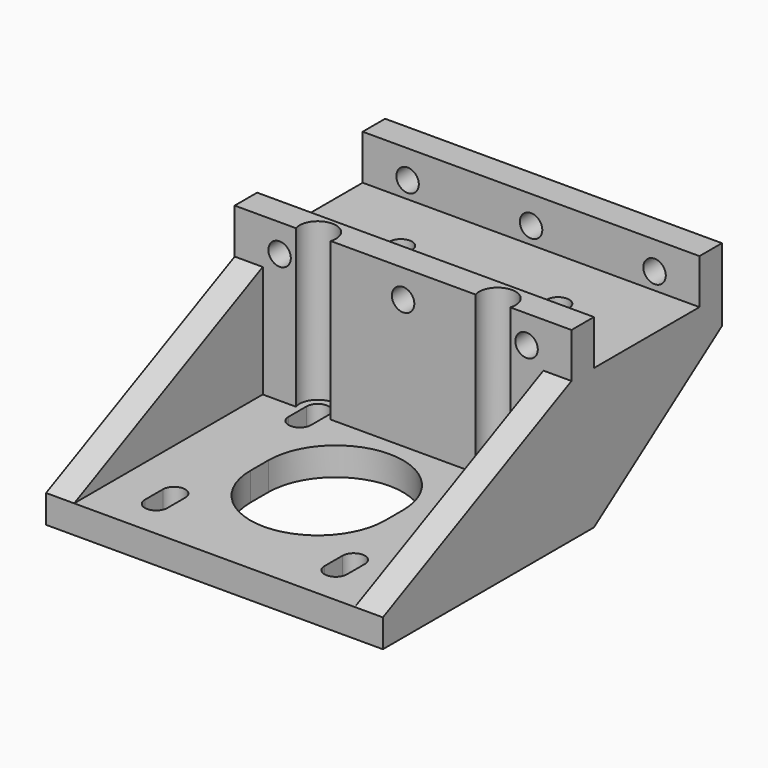
from build123d import *

# Parameters (mm, degrees)
F0_W           = 60
F0_H           = 47
F1_DEPTH       = 5
F3_DEPTH       = 20
F4_W           = 60
F4_H           = 5
F5_DEPTH       = 28.5
F7_DEPTH       = 5
F9_DEPTH       = 8
F10_W          = 60
F10_H          = 5
F11_DEPTH      = 8
F12_R          = 2
F13_DEPTH      = 25
F15_DEPTH      = 2.5
F15_DEPTH_BACK = 2.5
F16_R          = 2
F17_DEPTH      = 75.501
F18_R          = 3.25
F19_DEPTH      = 28
F20_DEPTH      = 138


# Not quite as in the source:
# - an extrude ends at something that could not be found from the text; its depth is read off the source's solid
# - a pattern or mirror of a feature is missing from the dataset's text; its kind, count and spacing are read off the source's solid
# - a feature names something its author has since deleted; it is built from what else it names


with BuildPart() as f1:
    # F0 (on Top) → F1 (new body)
    with BuildSketch(Plane.XY):
        with Locations((0, -1.5)):
            Rectangle(F0_W, F0_H)
        with BuildLine():
            Line((-14, -14), (-14, -18))
            ThreePointArc((-14, -18), (-16, -20), (-18, -18))
            Line((-18, -18), (-18, -14))
            ThreePointArc((-18, -14), (-16, -12), (-14, -14))
        make_face(mode=Mode.SUBTRACT)
        with BuildLine():
            Line((18, -14), (18, -18))
            ThreePointArc((18, -18), (16, -20), (14, -18))
            Line((14, -18), (14, -14))
            ThreePointArc((14, -14), (16, -12), (18, -14))
        make_face(mode=Mode.SUBTRACT)
        with BuildLine():
            ThreePointArc((-14, 14), (-16, 12), (-18, 14))
            Line((-18, 14), (-18, 18))
            ThreePointArc((-18, 18), (-16, 20), (-14, 18))
            Line((-14, 18), (-14, 14))
        make_face(mode=Mode.SUBTRACT)
        with BuildLine():
            Line((-12, -2), (-12, 2))
            ThreePointArc((-12, 2), (0, 14), (12, 2))
            Line((12, 2), (12, -2))
            ThreePointArc((12, -2), (0, -14), (-12, -2))
        make_face(mode=Mode.SUBTRACT)
        with BuildLine():
            Line((14, 14), (14, 18))
            ThreePointArc((14, 18), (16, 20), (18, 18))
            Line((18, 18), (18, 14))
            ThreePointArc((18, 14), (16, 12), (14, 14))
        make_face(mode=Mode.SUBTRACT)
    extrude(amount=F1_DEPTH)

    # F2 (on face) → F3 (join)
    with BuildSketch(Plane.XY.offset(5)):
        with BuildLine():
            Line((30, 22), (-30, 22))
            Line((-30, 22), (-30, 17))
            Line((-30, 17), (-18, 17))
            Line((-18, 17), (-18, 18))
            ThreePointArc((-18, 18), (-16, 20), (-14, 18))
            Line((-14, 18), (-14, 17))
            Line((-14, 17), (14, 17))
            Line((14, 17), (14, 18))
            ThreePointArc((14, 18), (16, 20), (18, 18))
            Line((18, 18), (18, 17))
            Line((18, 17), (30, 17))
            Line((30, 17), (30, 22))
        make_face()
    extrude(amount=F3_DEPTH)

    # F4 (on face) → F5 (join)
    with BuildSketch(Plane(origin=(0, 22, 0), x_dir=(-1, 0, 0), z_dir=(0, 1, 0))):
        with Locations((0, 22.5)):
            Rectangle(F4_W, F4_H)
    extrude(amount=F5_DEPTH)

    # F6 (on face) → F7 (join)
    with BuildSketch(Plane(origin=(-30, 0, 0), x_dir=(0, -1, 0), z_dir=(-1, 0, 0))):
        Polygon((-22, 20), (-50.5, 20), (-22, 0), align=None)
        Polygon((25, 5), (-17, 25), (-17, 5), align=None)
    f7 = extrude(amount=-F7_DEPTH)

    # F7_copies: F7 across plane
    add(f7.mirror(Plane(origin=(0, 0, 0), x_dir=(0, 0, 1), z_dir=(1, 0, 0))))

    # F8 (on face) → F9 (join)
    with BuildSketch(Plane.XY.offset(25)):
        with BuildLine():
            Line((30, 22), (-30, 22))
            Line((-30, 22), (-30, 17))
            Line((-30, 17), (-25, 17))
            Line((-25, 17), (-18, 17))
            Line((-18, 17), (-18, 18))
            ThreePointArc((-18, 18), (-16, 20), (-14, 18))
            Line((-14, 18), (-14, 17))
            Line((-14, 17), (14, 17))
            Line((14, 17), (14, 18))
            ThreePointArc((14, 18), (16, 20), (18, 18))
            Line((18, 18), (18, 17))
            Line((18, 17), (25, 17))
            Line((25, 17), (30, 17))
            Line((30, 17), (30, 22))
        make_face()
    extrude(amount=F9_DEPTH)

    # F10 (on face) → F11 (join)
    with BuildSketch(Plane.XY.offset(25)):
        with Locations((0, 48)):
            Rectangle(F10_W, F10_H)
    extrude(amount=F11_DEPTH)

    # F12 (on face) → F13 (cut)
    with BuildSketch(Plane.XY.offset(25)):
        with Locations((14, 34)):
            Circle(F12_R)
        with Locations((-14, 34)):
            Circle(F12_R)
    extrude(amount=-F13_DEPTH, mode=Mode.SUBTRACT)

    # F14 (on Right) → F15 (join, two sides)
    with BuildSketch(Plane.YZ) as f15_sk:
        Polygon((22, 20), (22, 0), (50.5, 20), align=None)
    extrude(amount=F15_DEPTH)
    extrude(f15_sk.sketch, amount=-F15_DEPTH_BACK)

    # F16 (on face) → F17 (cut, through all)
    with BuildSketch(Plane(origin=(0, 50.5, 0), x_dir=(-1, 0, 0), z_dir=(0, 1, 0))):
        with Locations((-22, 28)):
            Circle(F16_R)
        with Locations((22, 28)):
            Circle(F16_R)
        with Locations((0, 28)):
            Circle(F16_R)
    extrude(amount=-F17_DEPTH, mode=Mode.SUBTRACT)

    # F18 (on face) → F19 (cut, through all)
    with BuildSketch(Plane.XY.offset(33)):
        with Locations((-16, 18)):
            Circle(F18_R)
        with Locations((16, 18)):
            Circle(F18_R)
    extrude(amount=-F19_DEPTH, mode=Mode.SUBTRACT)

    # F16 (on face) → F20 (cut, through all)
    with BuildSketch(Plane(origin=(0, 50.5, 0), x_dir=(-1, 0, 0), z_dir=(0, 1, 0))):
        with Locations((-22, 28)):
            Circle(F16_R)
        with Locations((22, 28)):
            Circle(F16_R)
        with Locations((0, 28)):
            Circle(F16_R)
    extrude(amount=F20_DEPTH, mode=Mode.SUBTRACT)


solid = f1.part
